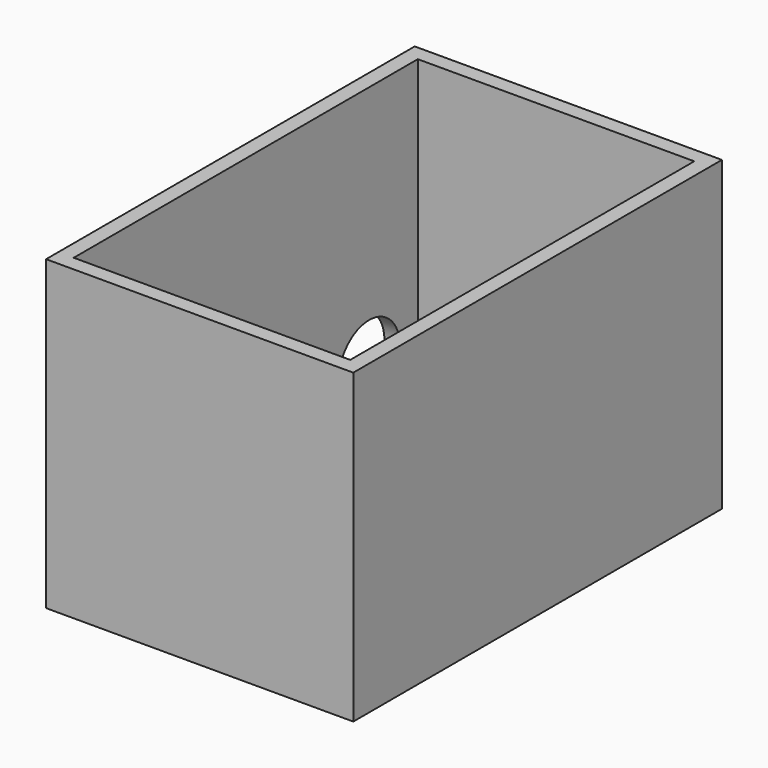
from build123d import *

# Parameters (mm, degrees)
F2_W     = 50.8
F2_H     = 76.2
F2_W_2   = 45.72
F2_H_2   = 71.12
F3_DEPTH = 50.8
F4_W     = 50.8
F4_H     = 76.2
F5_DEPTH = 2.54
F8_D     = 12.7
F8_DEPTH = 5.08
F8_TIP   = 3.8154649308


# Not quite as in the source:
# - a variable given as a bare number and used for a length is read in inches; the dataset says mm whatever the document's units were


with BuildPart() as f3:
    # F2 (on Top) → F3 (new body)
    with BuildSketch(Plane.XY):
        with Locations((25.4, 38.1)):
            Rectangle(F2_W, F2_H)
        with Locations((25.4, 38.1)):
            Rectangle(F2_W_2, F2_H_2, mode=Mode.SUBTRACT)
    extrude(amount=F3_DEPTH)

    # F4 (on Top) → F5 (join)
    with BuildSketch(Plane.XY):
        with Locations((25.4, 38.1)):
            Rectangle(F4_W, F4_H)
    extrude(amount=F5_DEPTH)

    # F8
    with Locations(Plane(origin=(0, 0, 0), x_dir=(0, -1, 0), z_dir=(-1, 0, 0))):
        with Locations((-14.4875170663, 10.56548208), (-32.958894968, 10.56548208), (-45.4774573445, 10.56548208), (-63.5905191302, 10.56548208)):
            Hole(F8_D / 2, depth=F8_DEPTH)
            with Locations((0, 0, -(F8_DEPTH + F8_TIP / 2))):  # 118° drill point
                Cone(0, F8_D / 2, F8_TIP, mode=Mode.SUBTRACT)


solid = f3.part
